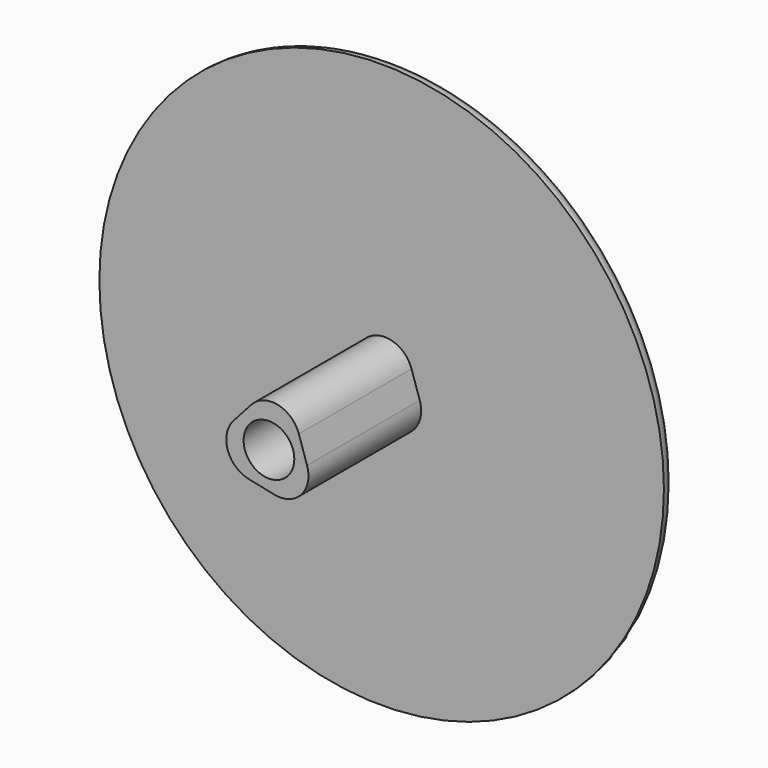
from build123d import *

# Parameters (mm, degrees)
F0_R     = 50.1
F0_R_2   = 4.5
F1_DEPTH = 3
F2_R     = 4.5
F3_DEPTH = 25
F4_R     = 2.99999
F5_R     = 5


# Not quite as in the source:
# - a fillet or chamfer is up to 0.001 mm smaller than in the source, because OpenCascade refuses the exact size


with BuildPart() as f1:
    # F0 (on Front) → F1 (new body)
    with BuildSketch(Plane.XZ):
        Circle(F0_R)
        Circle(F0_R_2, mode=Mode.SUBTRACT)
    extrude(amount=F1_DEPTH)

    # F2 (on face) → F3 (join)
    with BuildSketch(Plane.XZ.offset(3)):
        Polygon((9.4680966624, -8.46690492), (2.598506421, 12.4330646951), (-12.0666030834, -3.9661597751), align=None)
        Circle(F2_R, mode=Mode.SUBTRACT)
    extrude(amount=F3_DEPTH)

    # F4 (radius 3 in the source; OpenCascade refuses exactly that, so slightly less here)
    f4_edges = [f1.edges().sort_by_distance(p)[0] for p in [
        (-50.1, 0, 0),
    ]]
    fillet(f4_edges, radius=F4_R)

    # F5
    f5_edges = [f1.edges().sort_by_distance(p)[0] for p in [
        (2.598506, -15.5, 12.433065),
        (-12.066603, -15.5, -3.96616),
        (9.468097, -15.5, -8.466905),
    ]]
    fillet(f5_edges, radius=F5_R)


solid = f1.part
